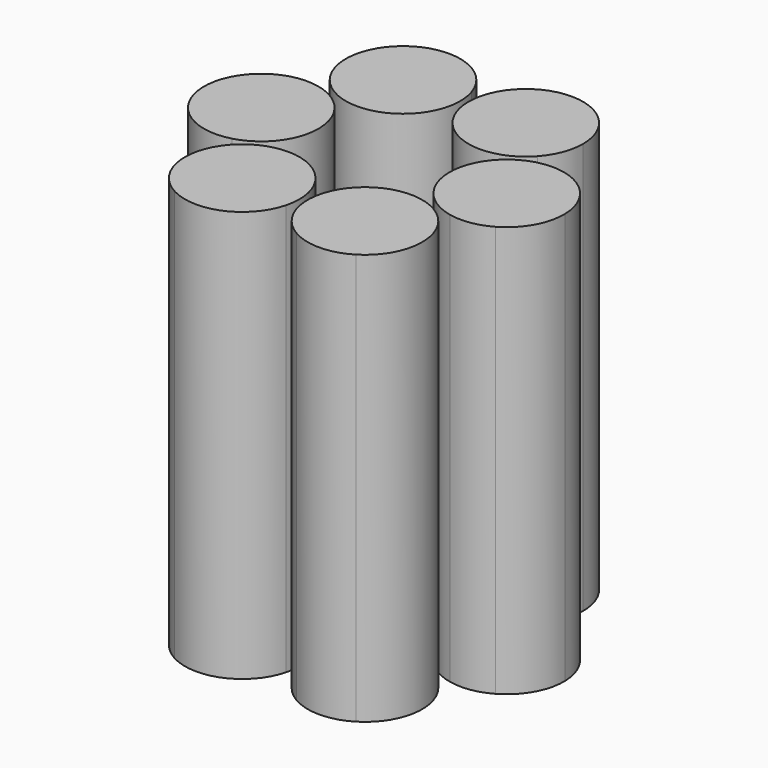
from build123d import *

# Parameters (mm, degrees)
F1_DEPTH = 65
F2_COUNT = 6


# Not quite as in the source:
# - a feature names something its author has since deleted; it is built from what else it names


with BuildPart() as f1:
    # F0 (on Top) → F1 (new body)
    with BuildSketch(Plane.XY):
        with BuildLine():
            ThreePointArc((0.294914085, 18.9977110643), (9.05, 16.7062114197), (15.7518514967, 10.6244611358))
            ThreePointArc((15.7518514967, 10.6244611358), (17.4925782805, 13.4465531589), (18.1, 16.7062114197))
            ThreePointArc((18.1, 16.7062114197), (16.8254084785, 21.3371425348), (13.3606579021, 24.6636436972))
            ThreePointArc((13.3606579021, 24.6636436972), (5.449453758, 25.0091366126), (0.294914085, 18.9977110643))
        make_face()
        with BuildLine():
            ThreePointArc((0.294914085, 18.9977110643), (4.7393421053, 8.7487791382), (15.7518514967, 10.6244611358))
            ThreePointArc((15.7518514967, 10.6244611358), (9.05, 16.7062114197), (0.294914085, 18.9977110643))
        make_face()
    extrude(amount=F1_DEPTH)


with BuildPart() as f2_1:
    # F2: instance of F1
    add(f1.part.rotate(Axis((0, 0, 0), (0, 0, 1)), 1 * 360 / F2_COUNT))


with BuildPart() as f2_2:
    # F2: instance of F1
    add(f1.part.rotate(Axis((0, 0, 0), (0, 0, 1)), 2 * 360 / F2_COUNT))


with BuildPart() as f2_3:
    # F2: instance of F1
    add(f1.part.rotate(Axis((0, 0, 0), (0, 0, 1)), 3 * 360 / F2_COUNT))


with BuildPart() as f2_4:
    # F2: instance of F1
    add(f1.part.rotate(Axis((0, 0, 0), (0, 0, 1)), 4 * 360 / F2_COUNT))


with BuildPart() as f2_5:
    # F2: instance of F1
    add(f1.part.rotate(Axis((0, 0, 0), (0, 0, 1)), 5 * 360 / F2_COUNT))


solid = Compound([f1.part, f2_1.part, f2_2.part, f2_3.part, f2_4.part, f2_5.part])
